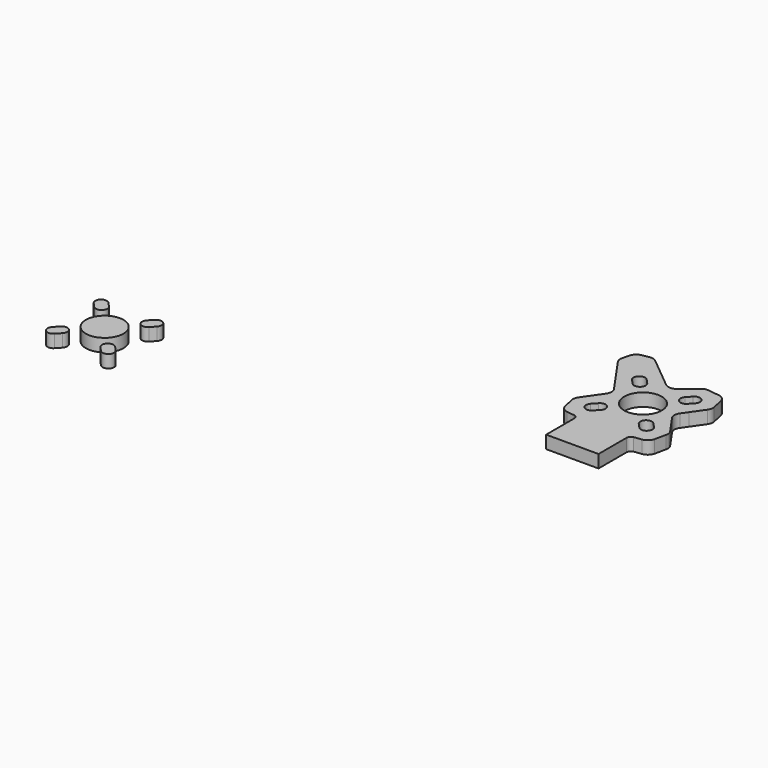
from build123d import *

# Parameters (mm, degrees)
F0_R     = 4.4142610292
F1_DEPTH = 3


with BuildPart() as f1:
    # F0 (on Top) → F1 (new body)
    with BuildSketch(Plane.XY):
        with BuildLine():
            Line((25.7442902372, 19.9449532418), (30.9231709689, 12.5199109316))
            Line((30.9231709689, 12.5199109316), (31.950624298, 11.0468350227))
            ThreePointArc((31.950624298, 11.0468350227), (32.3102271943, 9.9026771044), (31.950624298, 8.7585191861))
            Line((31.950624298, 8.7585191861), (30.9231709689, 7.2854432773))
            Line((30.9231709689, 7.2854432773), (28.9204229775, 4.4140721562))
            ThreePointArc((28.9204229775, 4.4140721562), (28.5999922268, 3.6638103222), (28.6058278806, 2.8480072634))
            Line((28.6058278806, 2.8480072634), (29.1742312803, 0.2141939336))
            ThreePointArc((29.1742312803, 0.2141939336), (29.7726093608, -0.8334562119), (30.8646685292, -1.3463245451))
            Line((30.8646685292, -1.3463245451), (32.6677180839, -1.5869417583))
            ThreePointArc((32.6677180839, -1.5869417583), (33.2878625229, -1.9194730277), (33.535440608, -2.5781544849))
            Line((33.535440608, -2.5781544849), (33.535440608, -10.8359819278))
            Line((33.535440608, -10.8359819278), (45.8317909572, -10.8359819278))
            Line((45.8317909572, -10.8359819278), (45.8317909572, -2.5781544849))
            ThreePointArc((45.8317909572, -2.5781544849), (46.0793690423, -1.9194730277), (46.6995134813, -1.5869417583))
            Line((46.6995134813, -1.5869417583), (48.502563036, -1.3463245451))
            ThreePointArc((48.502563036, -1.3463245451), (49.5946222044, -0.8334562119), (50.193000285, 0.2141939336))
            Line((50.193000285, 0.2141939336), (50.7614036847, 2.8480072634))
            ThreePointArc((50.7614036847, 2.8480072634), (50.7672393384, 3.6638103222), (50.4468085877, 4.4140721562))
            Line((50.4468085877, 4.4140721562), (48.4440605963, 7.2854432773))
            Line((48.4440605963, 7.2854432773), (47.4166072672, 8.7585191861))
            ThreePointArc((47.4166072672, 8.7585191861), (47.0570043709, 9.9026771044), (47.4166072672, 11.0468350227))
            Line((47.4166072672, 11.0468350227), (48.4440605963, 12.5199109316))
            Line((48.4440605963, 12.5199109316), (50.4468085877, 15.3912820527))
            ThreePointArc((50.4468085877, 15.3912820527), (50.7672393384, 16.1415438867), (50.7614036847, 16.9573469455))
            Line((50.7614036847, 16.9573469455), (50.193000285, 19.5911602753))
            ThreePointArc((50.193000285, 19.5911602753), (49.5946222044, 20.6388104208), (48.502563036, 21.151678754))
            Line((48.502563036, 21.151678754), (45.8317909572, 21.5080936584))
            ThreePointArc((45.8317909572, 21.5080936584), (45.0181238394, 21.4488103812), (44.2958246872, 21.0695313015))
            Line((44.2958246872, 21.0695313015), (41.5934278716, 18.844037405))
            Line((41.5934278716, 18.844037405), (40.9550271008, 18.3182978058))
            ThreePointArc((40.9550271008, 18.3182978058), (39.6836157826, 17.862160902), (38.4122044644, 18.3182978058))
            Line((38.4122044644, 18.3182978058), (37.7738036936, 18.844037405))
            Line((37.7738036936, 18.844037405), (30.7857099055, 24.5989139589))
            ThreePointArc((30.7857099055, 24.5989139589), (30.0266429494, 24.9883131973), (29.1743530908, 25.025948389))
            Line((29.1743530908, 25.025948389), (27.4730209089, 24.7324982196))
            ThreePointArc((27.4730209089, 24.7324982196), (26.4563522851, 24.2311578132), (25.8754814635, 23.2577378718))
            Line((25.8754814635, 23.2577378718), (25.4472023991, 21.5852483387))
            ThreePointArc((25.4472023991, 21.5852483387), (25.4167056377, 20.7326732053), (25.7442902372, 19.9449532418))
        make_face()
        with BuildLine():
            ThreePointArc((33.2652082458, 4.9401631557), (35.1728738329, 5.0163996805), (35.2491103578, 3.1087340934))
            Line((35.2491103578, 3.1087340934), (34.2316497676, 2.0065662534))
            ThreePointArc((34.2316497676, 2.0065662534), (32.3239841805, 1.9303297286), (32.2477476557, 3.8379953157))
            Line((32.2477476557, 3.8379953157), (33.2652082458, 4.9401631557))
        make_face(mode=Mode.SUBTRACT)
        with BuildLine():
            ThreePointArc((44.1181212074, 3.1087340934), (44.1943577323, 5.0163996805), (46.1020233194, 4.9401631557))
            Line((46.1020233194, 4.9401631557), (47.1194839096, 3.8379953157))
            ThreePointArc((47.1194839096, 3.8379953157), (47.0432473847, 1.9303297286), (45.1355817976, 2.0065662534))
            Line((45.1355817976, 2.0065662534), (44.1181212074, 3.1087340934))
        make_face(mode=Mode.SUBTRACT)
        with BuildLine():
            ThreePointArc((35.2491103578, 16.6966201155), (35.1728738329, 14.7889545284), (33.2652082458, 14.8651910532))
            Line((33.2652082458, 14.8651910532), (32.2477476557, 15.9673588932))
            ThreePointArc((32.2477476557, 15.9673588932), (32.3239841805, 17.8750244803), (34.2316497676, 17.7987879555))
            Line((34.2316497676, 17.7987879555), (35.2491103578, 16.6966201155))
        make_face(mode=Mode.SUBTRACT)
        with Locations((39.6836157826, 9.9026771044)):
            Circle(F0_R, mode=Mode.SUBTRACT)
        with BuildLine():
            Line((47.1194839096, 15.9673588932), (46.1020233194, 14.8651910532))
            ThreePointArc((46.1020233194, 14.8651910532), (44.1943577323, 14.7889545284), (44.1181212074, 16.6966201155))
            Line((44.1181212074, 16.6966201155), (45.1355817976, 17.7987879555))
            ThreePointArc((45.1355817976, 17.7987879555), (47.0432473847, 17.8750244803), (47.1194839096, 15.9673588932))
        make_face(mode=Mode.SUBTRACT)
    extrude(amount=F1_DEPTH)


with BuildPart() as f1b:
    # F0 (on Top) → F1, piece 2 (new body)
    with BuildSketch(Plane.XY):
        with BuildLine():
            Line((-63.8419478975, -21.8808193593), (-62.8244873074, -22.9829871993))
            ThreePointArc((-62.8244873074, -22.9829871993), (-60.9168217203, -23.0592237242), (-60.8405851954, -21.1515581371))
            Line((-60.8405851954, -21.1515581371), (-61.8580457856, -20.0493902971))
            ThreePointArc((-61.8580457856, -20.0493902971), (-63.7657113727, -19.9731537722), (-63.8419478975, -21.8808193593))
        make_face()
    extrude(amount=F1_DEPTH)


with BuildPart() as f1c:
    # F0 (on Top) → F1, piece 3 (new body)
    with BuildSketch(Plane.XY):
        with Locations((-56.4060797706, -27.9455011481)):
            Circle(F0_R)
    extrude(amount=F1_DEPTH)


with BuildPart() as f1d:
    # F0 (on Top) → F1, piece 4 (new body)
    with BuildSketch(Plane.XY):
        with BuildLine():
            ThreePointArc((-51.9715743458, -21.1515581371), (-51.8953378209, -23.0592237242), (-49.9876722338, -22.9829871993))
            Line((-49.9876722338, -22.9829871993), (-48.9702116437, -21.8808193593))
            ThreePointArc((-48.9702116437, -21.8808193593), (-49.0464481685, -19.9731537722), (-50.9541137556, -20.0493902971))
            Line((-50.9541137556, -20.0493902971), (-51.9715743458, -21.1515581371))
        make_face()
    extrude(amount=F1_DEPTH)


with BuildPart() as f1e:
    # F0 (on Top) → F1, piece 5 (new body)
    with BuildSketch(Plane.XY):
        with BuildLine():
            Line((-48.9702116437, -34.0101829368), (-49.9876722338, -32.9080150968))
            ThreePointArc((-49.9876722338, -32.9080150968), (-51.8953378209, -32.831778572), (-51.9715743458, -34.7394441591))
            Line((-51.9715743458, -34.7394441591), (-50.9541137556, -35.8416119991))
            ThreePointArc((-50.9541137556, -35.8416119991), (-49.0464481685, -35.9178485239), (-48.9702116437, -34.0101829368))
        make_face()
    extrude(amount=F1_DEPTH)


with BuildPart() as f1f:
    # F0 (on Top) → F1, piece 6 (new body)
    with BuildSketch(Plane.XY):
        with BuildLine():
            Line((-61.8580457856, -35.8416119991), (-60.8405851954, -34.7394441591))
            ThreePointArc((-60.8405851954, -34.7394441591), (-60.9168217203, -32.831778572), (-62.8244873074, -32.9080150968))
            Line((-62.8244873074, -32.9080150968), (-63.8419478975, -34.0101829368))
            ThreePointArc((-63.8419478975, -34.0101829368), (-63.7657113727, -35.9178485239), (-61.8580457856, -35.8416119991))
        make_face()
    extrude(amount=F1_DEPTH)


solid = Compound([f1.part, f1b.part, f1c.part, f1d.part, f1e.part, f1f.part])
